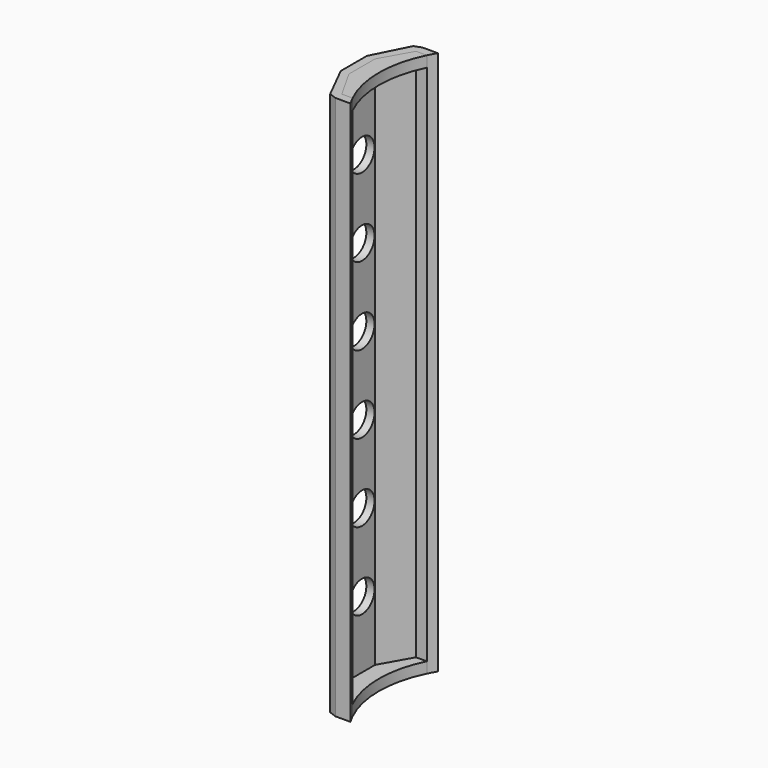
from build123d import *
from build123d import SkipClean  # not in build123d's __all__

# Parameters (mm, degrees)
F1_DEPTH = 99.8
F2_R     = 2.875
F3_DEPTH = 4
F4_DEPTH = 2
F6_DEPTH = 2


with BuildPart() as f1:
    # F0 (on Top) → F1 (new body)
    with BuildSketch(Plane.XY):
        with BuildLine():
            ThreePointArc((-17.2717254494, 8.5), (-16.8769277982, 9.2591472661), (-16.4487841496, 10))
            Line((-16.4487841496, 10), (-19.25, 10))
            Line((-19.25, 10), (-20.572897503, 9.5070659068))
            Line((-20.572897503, 9.5070659068), (-23.85, 3))
            Line((-23.85, 3), (-23.85, -3))
            Line((-23.85, -3), (-20.572897503, -9.5070659068))
            Line((-20.572897503, -9.5070659068), (-19.25, -10))
            Line((-19.25, -10), (-16.4487841496, -10))
            ThreePointArc((-16.4487841496, -10), (-16.8769277982, -9.2591472661), (-17.2717254494, -8.5))
            Line((-17.2717254494, -8.5), (-19.25, -8.5))
            Line((-19.25, -8.5), (-22.35, -3))
            Line((-22.35, -3), (-22.35, 0))
            Line((-22.35, 0), (-22.35, 3))
            Line((-22.35, 3), (-19.25, 8.5))
            Line((-19.25, 8.5), (-17.2717254494, 8.5))
        make_face()
    extrude(amount=F1_DEPTH)

    # F2 (on face) → F3 (cut)
    with BuildSketch(Plane(origin=(-23.85, 0, 0), x_dir=(0, -1, 0), z_dir=(-1, 0, 0))):
        with Locations((0, 14.26)):
            Circle(F2_R)
        with Locations((0, 28.52)):
            Circle(F2_R)
        with Locations((0, 42.78)):
            Circle(F2_R)
        with Locations((0, 57.04)):
            Circle(F2_R)
        with Locations((0, 71.3)):
            Circle(F2_R)
        with Locations((0, 85.56)):
            Circle(F2_R)
    extrude(amount=-F3_DEPTH, mode=Mode.SUBTRACT)

    # F0 (on Top) → F4 (join)
    with BuildSketch(Plane.XY):
        with BuildLine():
            ThreePointArc((-17.2717254494, -8.5), (-19.25, 0), (-17.2717254494, 8.5))
            Line((-17.2717254494, 8.5), (-19.25, 8.5))
            Line((-19.25, 8.5), (-22.35, 3))
            Line((-22.35, 3), (-22.35, 0))
            Line((-22.35, 0), (-22.35, -3))
            Line((-22.35, -3), (-19.25, -8.5))
            Line((-19.25, -8.5), (-17.2717254494, -8.5))
        make_face()
    extrude(amount=F4_DEPTH)

    # F5 (on face) → F6 (join)
    with BuildSketch(Plane.XY.offset(99.8)):
        with BuildLine():
            ThreePointArc((-17.2717254494, -8.5), (-19.25, 0), (-17.2717254494, 8.5))
            Line((-17.2717254494, 8.5), (-19.25, 8.5))
            Line((-19.25, 8.5), (-22.35, 3))
            Line((-22.35, 3), (-22.35, -3))
            Line((-22.35, -3), (-19.25, -8.5))
            Line((-19.25, -8.5), (-17.2717254494, -8.5))
        make_face()
    with SkipClean():  # cleaning this boolean's faces spoils the solid; the shape is the same uncleaned
        extrude(amount=-F6_DEPTH)


solid = f1.part
